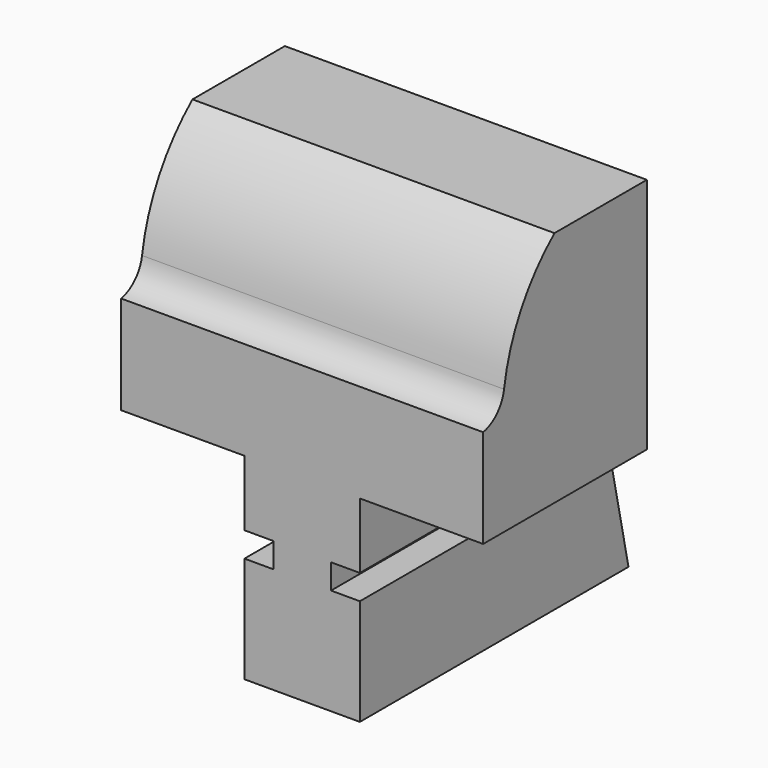
from build123d import *

# Parameters (mm, degrees)
F0_W          = 65.024
F0_H          = 84.074
F1_DEPTH      = 35.052
F1_DEPTH_BACK = 35.052
F3_DEPTH      = 63.5
F4_W          = 77.3881527235
F4_H          = 70.5238262352
F5_DEPTH      = 38.1
F7_DEPTH      = 25.4
F9_DEPTH      = 38.1
F10_T1_DEPTH  = 70.104


# Not quite as in the source:
# - a fillet or chamfer that OpenCascade refuses, or shapes differently, is made with other operations: its cross-section is extruded or revolved along the edge and cut away or added


with BuildPart() as f1:
    # F0 (on Right) → F1 (new body, two sides)
    with BuildSketch(Plane.YZ) as f1_sk:
        Rectangle(F0_W, F0_H)
    extrude(amount=F1_DEPTH)
    extrude(f1_sk.sketch, amount=-F1_DEPTH_BACK)

    # F2 (on Front) → F3 (cut, symmetric)
    with BuildSketch(Plane.XZ):
        Polygon((-11.176, -16.637), (-11.176, -3.937), (-78.232, -3.937), (-78.232, -87.8102174824), (-11.176, -87.8102174824), (-11.176, -21.463), (-5.588, -21.463), (-5.588, -16.637), align=None)
        Polygon((75.6774835046, -3.937), (11.176, -3.937), (11.176, -16.637), (5.588, -16.637), (5.588, -21.463), (11.176, -21.463), (11.176, -87.8102174824), (75.6774835046, -87.8102174824), align=None)
    extrude(amount=F3_DEPTH, both=True, mode=Mode.SUBTRACT)

    # F4 (on Right) → F5 (cut, symmetric)
    with BuildSketch(Plane.YZ):
        with Locations((45.8060763618, 28.2769131176)):
            Rectangle(F4_W, F4_H)
    extrude(amount=F5_DEPTH, both=True, mode=Mode.SUBTRACT)

    # F6 (on face) → F7 (cut, symmetric)
    with BuildSketch(Plane.YZ.offset(11.176)):
        Polygon((32.512, -21.463), (32.512, -42.037), (58.1510797716, -47.1596371092), (55.1210400309, 2.9251785083), (22.86, 2.9251785083), (28.0953935412, -21.463), align=None)
        Polygon((28.0953935412, -21.463), (32.512, -42.037), (32.512, -21.463), align=None)
    extrude(amount=F7_DEPTH, both=True, mode=Mode.SUBTRACT)

    # F8 (on Right) → F9 (cut, symmetric)
    with BuildSketch(Plane.YZ):
        with BuildLine():
            ThreePointArc((-27.8538692881, 15.113), (-17.5873761822, 39.8985068942), (7.1981307119, 50.165))
            Line((7.1981307119, 50.165), (-30.8227688074, 66.0536216443))
            Line((-30.8227688074, 66.0536216443), (-47.4338419735, 15.113))
            Line((-47.4338419735, 15.113), (-27.8538692881, 15.113))
        make_face()
    extrude(amount=F9_DEPTH, both=True, mode=Mode.SUBTRACT)

    # F10: fillet of radius 6.35 on 1 edges, made by hand

    # F10_s2 → F10_t1 (join)
    with BuildSketch(Plane.YZ.offset(-35.052)):
        with BuildLine():
            ThreePointArc((-32.512, 15.113), (-29.1481831988, 16.9504285484), (-27.454542127, 20.3888856242))
            ThreePointArc((-27.454542127, 20.3888856242), (-27.7538949257, 17.7584882017), (-27.8538692881, 15.113))
            Line((-27.8538692881, 15.113), (-32.512, 15.113))
        make_face()
    extrude(amount=F10_T1_DEPTH)


solid = f1.part
